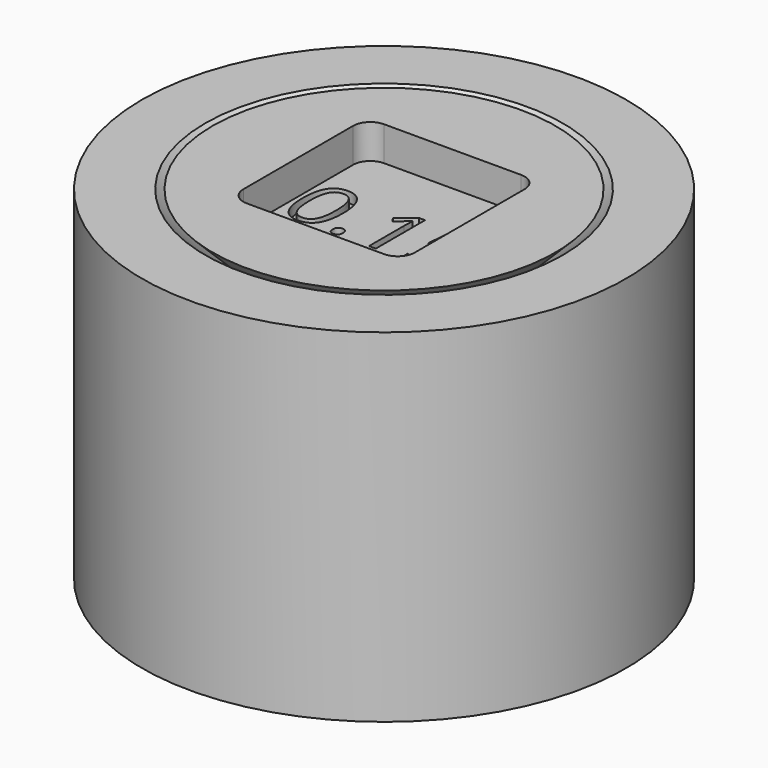
from build123d import *

# Parameters (mm, degrees)
F4_DEPTH     = 1
F5_TEXT_SIZE = 2.514339593
F6_DEPTH     = 1.3


# Not quite as in the source:
# - Text() gives the source's letters only with a copy of the font that has no kerning and outlines rounded to 1/6400 em; it was checked with that copy


with BuildPart() as f1:
    # F0 (on Front) → F1 (revolve)
    with BuildSketch(Plane.XZ):
        with BuildLine():
            Line((-5, 0), (0, 0))
            Line((0, 0), (0, 10))
            Line((0, 10), (-5, 10))
            Line((-5, 10), (-2.7928932188, 7.7928932188))
            ThreePointArc((-2.7928932188, 7.7928932188), (-2.5761204675, 7.46846987), (-2.5, 7.0857864376))
            Line((-2.5, 7.0857864376), (-2.5, 2.9142135624))
            ThreePointArc((-2.5, 2.9142135624), (-2.5761204675, 2.53153013), (-2.7928932188, 2.2071067812))
            Line((-2.7928932188, 2.2071067812), (-5, 0))
        make_face()
    revolve(axis=Axis((0, 0, 5), (0, 0, 1)))

    # F3 (on face) → F4 (cut)
    with BuildSketch(Plane.XY.offset(10)):
        with BuildLine():
            Line((2, 2.5), (-2, 2.5))
            ThreePointArc((-2, 2.5), (-2.3535533906, 2.3535533906), (-2.5, 2))
            Line((-2.5, 2), (-2.5, -2))
            ThreePointArc((-2.5, -2), (-2.3535533906, -2.3535533906), (-2, -2.5))
            Line((-2, -2.5), (2, -2.5))
            ThreePointArc((2, -2.5), (2.3535533906, -2.3535533906), (2.5, -2))
            Line((2.5, -2), (2.5, 2))
            ThreePointArc((2.5, 2), (2.3535533906, 2.3535533906), (2, 2.5))
        make_face()
    extrude(amount=-F4_DEPTH, mode=Mode.SUBTRACT)

    # F5 (on offset) → F6 (cut)
    with BuildSketch(Plane.XY.offset(10)):
        with Locations((-2.5, -0.9051622535)):
            Text('0.15', F5_TEXT_SIZE, font='Open Sans', text_align=(TextAlign.LEFT, TextAlign.BOTTOM))
    extrude(amount=-F6_DEPTH, mode=Mode.SUBTRACT)


with BuildPart() as f1b:
    # F0 (on Front) → F1, piece 2 (revolve)
    with BuildSketch(Plane.XZ):
        with BuildLine():
            Line((-7.0621320344, 10), (-7.0621320344, 0))
            Line((-7.0621320344, 0), (-5.2121320344, 0))
            Line((-5.2121320344, 0), (-2.9428932188, 2.2692388155))
            ThreePointArc((-2.9428932188, 2.2692388155), (-2.7261204675, 2.5936621644), (-2.65, 2.9763455967))
            Line((-2.65, 2.9763455967), (-2.65, 7.0236544033))
            ThreePointArc((-2.65, 7.0236544033), (-2.7261204675, 7.4063378356), (-2.9428932188, 7.7307611845))
            Line((-2.9428932188, 7.7307611845), (-5.2121320344, 10))
            Line((-5.2121320344, 10), (-7.0621320344, 10))
        make_face()
    revolve(axis=Axis((0, 0, 5), (0, 0, 1)))


solid = Compound([f1.part, f1b.part])
